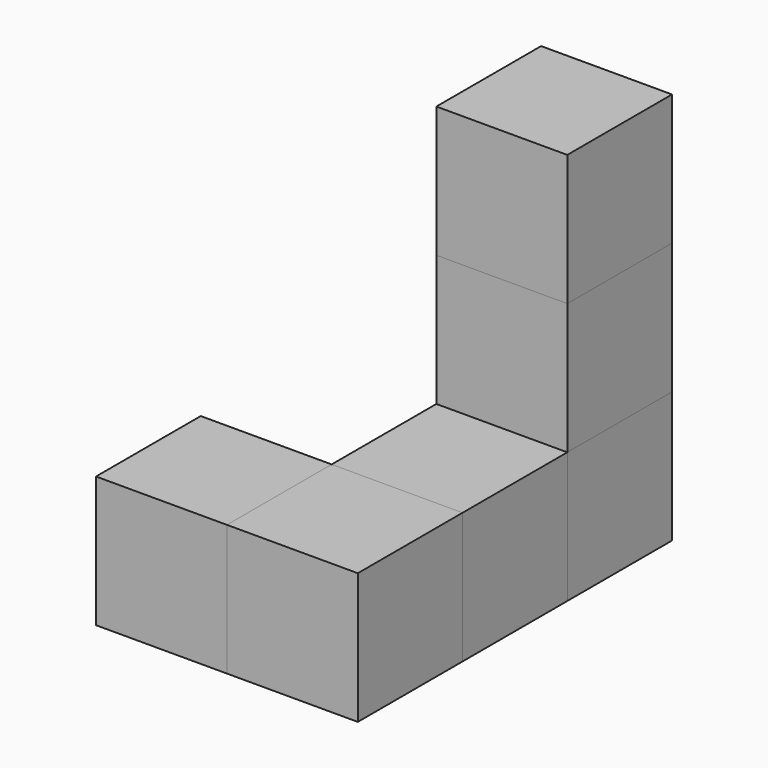
from build123d import *

# Parameters (mm, degrees)
F0_W     = 12.7
F0_H     = 12.7
F1_DEPTH = 12.7


with BuildPart() as f1:
    # F0 (on Front) → F1 (new body)
    with BuildSketch(Plane.XZ):
        with Locations((-26.4234156107, -11.7347757367)):
            Rectangle(F0_W, F0_H)
    extrude(amount=F1_DEPTH)


with BuildPart() as f2_1:
    # F2: copy of F1
    add(f1.part.moved(Location((0, 12.7, 0))))


with BuildPart() as f3_1:
    # F3: copy of F2_1
    add(f2_1.part.moved(Location((0, 12.7, 0))))


with BuildPart() as f4_1:
    # F4: copy of F1
    add(f1.part.moved(Location((-12.7, 0, 0))))


with BuildPart() as f5_1:
    # F5: copy of F3_1
    add(f3_1.part.moved(Location((0, 0, 12.7))))


with BuildPart() as f6_1:
    # F6: copy of F5_1
    add(f5_1.part.moved(Location((0, 0, 12.7))))


solid = Compound([f1.part, f2_1.part, f3_1.part, f4_1.part, f5_1.part, f6_1.part])
